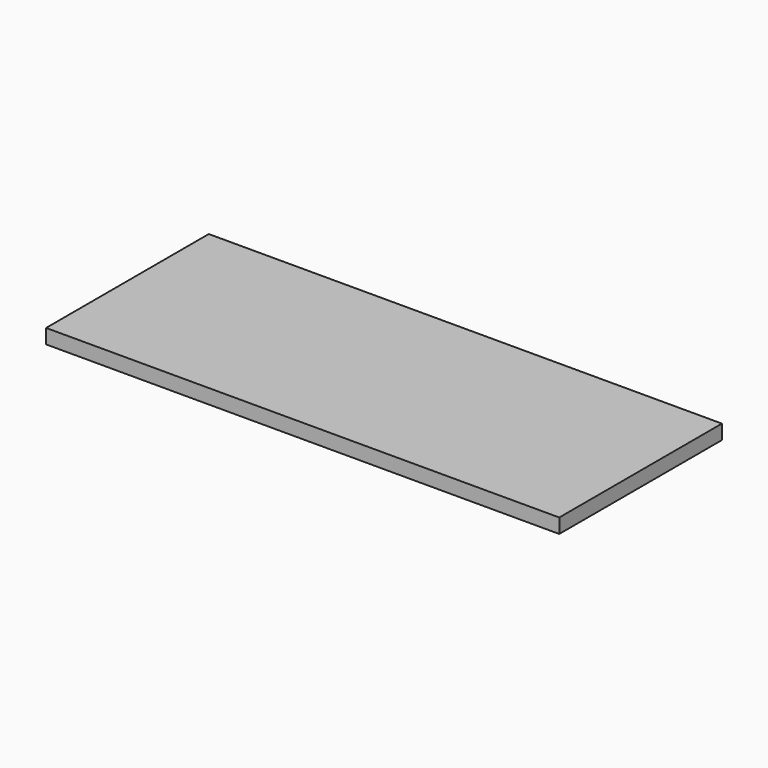
from build123d import *

# Parameters (mm, degrees)
F0_W     = 673.1
F0_H     = 266.7
F1_DEPTH = 19.05


# Not quite as in the source:
# - a length typed as a fraction of an inch, garbled in the dataset ("3 / 203.2 mm" for 3/8 in), is restored


with BuildPart() as f1:
    # F0 (on Top) → F1 (new body)
    with BuildSketch(Plane.XY):
        Rectangle(F0_W, F0_H)
    extrude(amount=F1_DEPTH)


solid = f1.part
